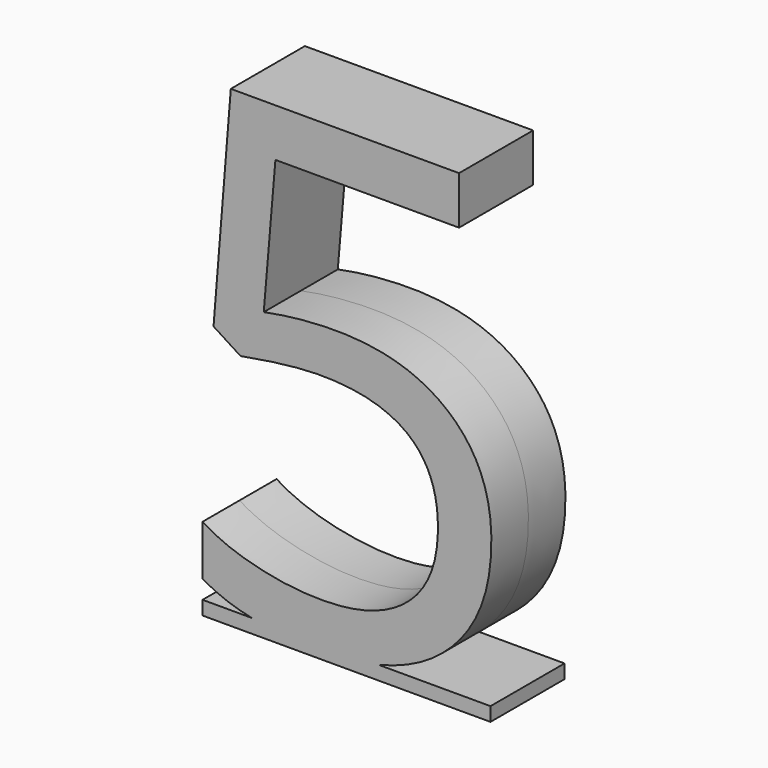
from build123d import *

# Parameters (mm, degrees)
F0_TEXT_SIZE  = 138.8888888889
F1_DEPTH      = 10
F1_DEPTH_BACK = 10
F2_W          = 62.1944444444
F2_H          = 20
F3_DEPTH      = 3


# Not quite as in the source:
# - Text() gives the source's letters only with a copy of the font that has no kerning and outlines rounded to 1/6400 em; it was checked with that copy


with BuildPart() as f1:
    # F0 (on Front) → F1 (new body, two sides)
    with BuildSketch(Plane.XZ) as f1_sk:
        with Locations((-40.2126736111, 0)):
            Text('5', F0_TEXT_SIZE, font='Open Sans', text_align=(TextAlign.LEFT, TextAlign.BOTTOM))
    extrude(amount=F1_DEPTH)
    extrude(f1_sk.sketch, amount=-F1_DEPTH_BACK)

    # F2 (on Top) → F3 (join)
    with BuildSketch(Plane.XY):
        with Locations((-0.0876736111, 0)):
            Rectangle(F2_W, F2_H)
    extrude(amount=-F3_DEPTH)


solid = f1.part
